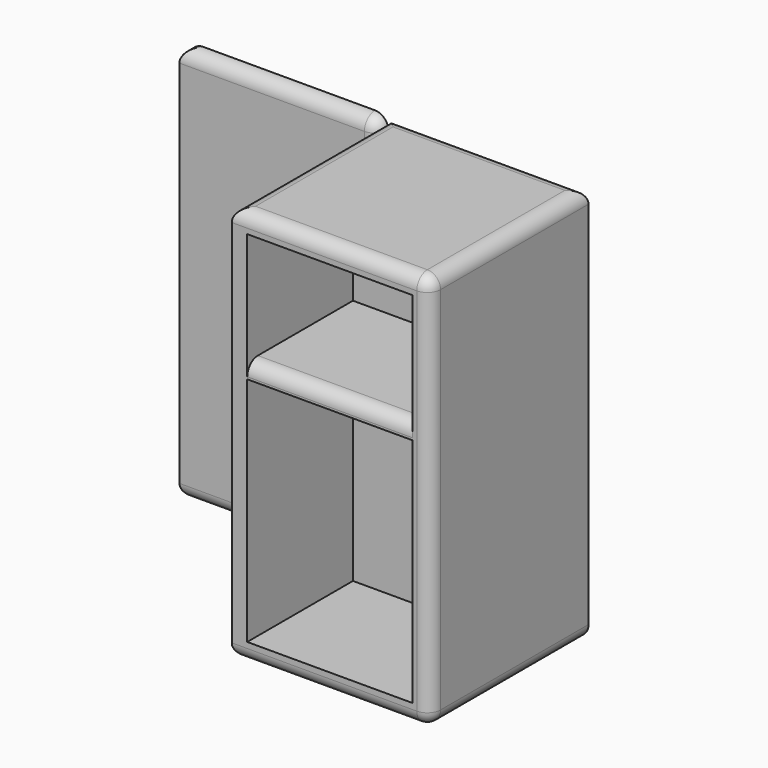
from build123d import *

# Parameters (mm, degrees)
F0_W     = 76.2
F0_H     = 152.4
F1_DEPTH = 5.08
F0_W_2   = 63.5
F0_H_2   = 88.9
F0_H_3   = 43.18
F2_DEPTH = 76.2
F3_DEPTH = 25.4
F4_R     = 5.07999
F4_2_R   = 5.07999


# Not quite as in the source:
# - a fillet or chamfer is up to 0.001 mm smaller than in the source, because OpenCascade refuses the exact size


with BuildPart() as f1:
    # F0 (on Front) → F1 (new body)
    with BuildSketch(Plane.XZ):
        with Locations((-38.910630511, -0.5404228303)):
            Rectangle(F0_W, F0_H)
    extrude(amount=F1_DEPTH)

    # F4 (radius 5.08 in the source; OpenCascade refuses exactly that, so slightly less here)
    f4_edges = [f1.edges().sort_by_distance(p)[0] for p in [
        (-0.810631, -5.08, -0.540423),
        (-38.910631, -5.08, -76.740423),
        (-77.010631, -2.54, 75.659577),
        (-77.010631, -2.54, -76.740423),
        (-0.810631, -2.54, 75.659577),
        (-38.910631, -5.08, 75.659577),
        (-0.810631, -2.54, -76.740423),
    ]]
    fillet(f4_edges, radius=F4_R)


with BuildPart() as f2:
    # F0 (on Front) → F2 (new body)
    with BuildSketch(Plane.XZ):
        with Locations((38.1, -0.5404228303)):
            Rectangle(F0_W, F0_H)
        with Locations((37.6946805432, -24.9946735409)):
            Rectangle(F0_W_2, F0_H_2, mode=Mode.SUBTRACT)
        with Locations((37.6946805432, 46.99)):
            Rectangle(F0_W_2, F0_H_3, mode=Mode.SUBTRACT)
    extrude(amount=F2_DEPTH)

    # F0 (on Front) → F3 (join)
    with BuildSketch(Plane.XZ):
        with Locations((37.6946805432, 46.99)):
            Rectangle(F0_W_2, F0_H_3)
        with Locations((37.6946805432, -24.9946735409)):
            Rectangle(F0_W_2, F0_H_2)
    extrude(amount=F3_DEPTH)

    # F4#2 (radius 5.08 in the source; OpenCascade refuses exactly that, so slightly less here)
    f4_2_edges = [f2.edges().sort_by_distance(p)[0] for p in [
        (76.2, -76.2, -0.540423),
        (38.1, 0, 75.659577),
        (37.694681, -76.2, 25.4),
        (38.1, -76.2, -76.740423),
        (38.1, -76.2, 75.659577),
        (76.2, -38.1, 75.659577),
        (0, -38.1, 75.659577),
        (76.2, -38.1, -76.740423),
        (0, -38.1, -76.740423),
    ]]
    fillet(f4_2_edges, radius=F4_2_R)


solid = Compound([f1.part, f2.part])
